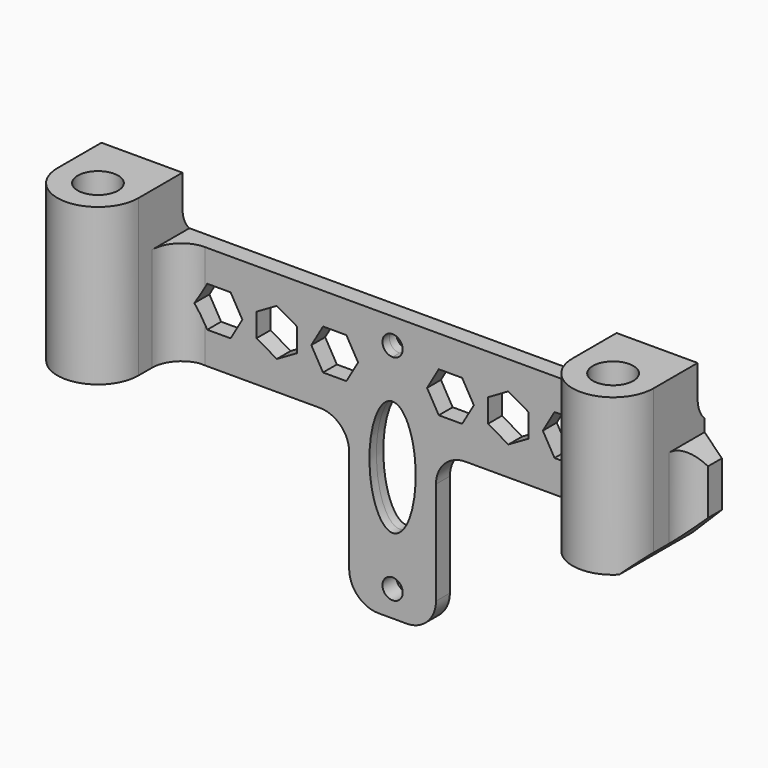
from build123d import *

# Parameters (mm, degrees)
F1_DEPTH      = 1.5
F2_R          = 3.5
F3_DEPTH      = 9
F4_DEPTH      = 9
F5_W          = 7.5
F5_H          = 37
F6_DEPTH      = 1.5
F8_DEPTH      = 12.7
F9_T1_DEPTH   = 3
F9_T3_DEPTH   = 17.9406090155
F9_T5_DEPTH   = 17.9406090155
F9_T7_DEPTH   = 17.9406090155
F9_T9_DEPTH   = 17.9406090155
F9_T11_DEPTH  = 14
F9_T13_DEPTH  = 14
F9_T15_DEPTH  = 3
F9_T17_DEPTH  = 28.4
F9_T19_DEPTH  = 28.4
F10_T1_DEPTH  = 29.1282991577
F10_T6_DEPTH  = 29.1282991577
F10_T11_DEPTH = 29.1282991577
F12_DEPTH     = 5.0038


# Not quite as in the source:
# - a fillet or chamfer that OpenCascade refuses, or shapes differently, is made with other operations: its cross-section is extruded or revolved along the edge and cut away or added


with BuildPart() as f1:
    # F0 (on Front) → F1 (new body, symmetric)
    with BuildSketch(Plane.XZ):
        Polygon((-54.5, 8.9406090155), (-54.5, -0.0593909845), (-54.5, -9.0593909845), (0, -9.0593909845), (0, 8.9406090155), align=None)
        Polygon((54.5, 8.9406090155), (0, 8.9406090155), (0, -9.0593909845), (54.5, -9.0593909845), (54.5, -0.0593909845), align=None)
    extrude(amount=F1_DEPTH, both=True)

    # F2 (on Top) → F3 (join, symmetric)
    with BuildSketch(Plane.XY):
        with BuildLine():
            ThreePointArc((-51.5, -9.5), (-44.5, -16.5), (-37.5, -9.5))
            ThreePointArc((-37.5, -9.5), (-44.5, -2.5), (-51.5, -9.5))
        make_face()
        with Locations((-44.5, -9.5)):
            Circle(F2_R, mode=Mode.SUBTRACT)
        with BuildLine():
            ThreePointArc((-51.5, -9.5), (-44.5, -2.5), (-37.5, -9.5))
            Line((-37.5, -9.5), (-37.5, 0))
            Line((-37.5, 0), (-51.5, 0))
            Line((-51.5, 0), (-51.5, -9.5))
        make_face()
        with BuildLine():
            Line((37.5, 0), (37.5, -9.5))
            ThreePointArc((37.5, -9.5), (44.5, -2.5), (51.5, -9.5))
            Line((51.5, -9.5), (51.5, 0))
            Line((51.5, 0), (37.5, 0))
        make_face()
        with BuildLine():
            ThreePointArc((51.5, -9.5), (44.5, -2.5), (37.5, -9.5))
            ThreePointArc((37.5, -9.5), (44.5, -16.5), (51.5, -9.5))
        make_face()
        with Locations((44.5, -9.5)):
            Circle(F2_R, mode=Mode.SUBTRACT)
    extrude(amount=F3_DEPTH, both=True)

    # F4 (add): faces of the model
    f4_faces = [f1.faces().sort_by_distance(p)[0] for p in [
        (-44.5, -16.2836091499, 9),
        (37.7163908501, -4.75, 9),
    ]]
    extrude(f4_faces, amount=F4_DEPTH)

    # F5 (on Front) → F6 (join, symmetric)
    with BuildSketch(Plane.XZ):
        with Locations((3.75, -18.5)):
            Rectangle(F5_W, F5_H)
        with Locations((-3.75, -18.5)):
            Rectangle(F5_W, F5_H)
    extrude(amount=F6_DEPTH, both=True)

    # F7 (on Front) → F8 (cut, symmetric)
    with BuildSketch(Plane.XZ):
        with BuildLine():
            ThreePointArc((1.75, -32.5), (1.2374368671, -31.2625631329), (0, -30.75))
            ThreePointArc((0, -30.75), (-1.2374368671, -33.7374368671), (1.75, -32.5))
        make_face()
        with BuildLine():
            add(Edge.make_bspline(
                [(0, -24), (4, -24), (4, -14), (4, -4), (0, -4)],
                knots=[0, 0, 0, 1.5707963268, 1.5707963268, 3.1415926536, 3.1415926536, 3.1415926536], degree=2, weights=[1, 0.7071067812, 1, 0.7071067812, 1]))
            Line((0, -4), (0, -14))
            Line((0, -14), (0, -24))
        make_face()
        with BuildLine():
            Line((0, -14), (0, -4))
            add(Edge.make_bspline(
                [(0, -4), (-4, -4), (-4, -14), (-4, -24), (0, -24)],
                knots=[3.1415926536, 3.1415926536, 3.1415926536, 4.7123889804, 4.7123889804, 6.2831853072, 6.2831853072, 6.2831853072], degree=2, weights=[1, 0.7071067812, 1, 0.7071067812, 1]))
            Line((0, -24), (0, -14))
        make_face()
        with BuildLine():
            ThreePointArc((1.75, 4.5), (-1.2374368671, 5.7374368671), (0, 2.75))
            ThreePointArc((0, 2.75), (1.2374368671, 3.2625631329), (1.75, 4.5))
        make_face()
    extrude(amount=F8_DEPTH, both=True, mode=Mode.SUBTRACT)

    # F9: fillet of radius 5.08 on 10 edges, made by hand

    # F9_s2 → F9_t1 (join)
    with BuildSketch(Plane.XZ.offset(-1.5)):
        with BuildLine():
            ThreePointArc((-12.58, -9.0593909845), (-8.9878975516, -10.547288536), (-7.5, -14.1393909845))
            Line((-7.5, -14.1393909845), (-7.3984, -14.1393909845))
            Line((-7.3984, -14.1393909845), (-7.3984, -8.9577909845))
            Line((-7.3984, -8.9577909845), (-12.58, -8.9577909845))
            Line((-12.58, -8.9577909845), (-12.58, -9.0593909845))
        make_face()
    extrude(amount=F9_T1_DEPTH)

    # F9_s4 → F9_t3 (join)
    with BuildSketch(Plane.XY.offset(-9)):
        with BuildLine():
            ThreePointArc((-54.5, -1.5), (-52.3154484409, -3.3742173421), (-51.5, -6.1346520905))
            Line((-51.5, -6.1346520905), (-51.3984, -6.1346520905))
            Line((-51.3984, -6.1346520905), (-51.3984, -1.5))
            Line((-51.3984, -1.5), (-51.5, -1.3984))
            ThreePointArc((-51.5, -1.3984), (-53, -1.3984), (-54.4584, -1.4073069582))
            Line((-54.4584, -1.4073069582), (-54.5, -1.5))
        make_face()
    extrude(amount=F9_T3_DEPTH)

    # F9_s6 → F9_t5 (join)
    with BuildSketch(Plane.XY.offset(-9)):
        with BuildLine():
            ThreePointArc((-32.42, -1.5), (-36.0121024484, -2.9878975516), (-37.5, -6.58))
            Line((-37.5, -6.58), (-37.6016, -6.58))
            Line((-37.6016, -6.58), (-37.6016, -1.3984))
            Line((-37.6016, -1.3984), (-32.42, -1.3984))
            Line((-32.42, -1.3984), (-32.42, -1.5))
        make_face()
    extrude(amount=F9_T5_DEPTH)

    # F9_s8 → F9_t7 (join)
    with BuildSketch(Plane.XY.offset(-9)):
        with BuildLine():
            ThreePointArc((32.42, -1.5), (36.0121024484, -2.9878975516), (37.5, -6.58))
            Line((37.5, -6.58), (37.6016, -6.58))
            Line((37.6016, -6.58), (37.6016, -1.3984))
            Line((37.6016, -1.3984), (32.42, -1.3984))
            Line((32.42, -1.3984), (32.42, -1.5))
        make_face()
    extrude(amount=F9_T7_DEPTH)

    # F9_s10 → F9_t9 (join)
    with BuildSketch(Plane.XY.offset(-9)):
        with BuildLine():
            ThreePointArc((54.5, -1.5), (52.3154484409, -3.3742173421), (51.5, -6.1346520905))
            Line((51.5, -6.1346520905), (51.3984, -6.1346520905))
            Line((51.3984, -6.1346520905), (51.3984, -1.5))
            Line((51.3984, -1.5), (51.5, -1.3984))
            ThreePointArc((51.5, -1.3984), (53, -1.3984), (54.4584, -1.4073069582))
            Line((54.4584, -1.4073069582), (54.5, -1.5))
        make_face()
    extrude(amount=F9_T9_DEPTH)

    # F9_s12 → F9_t11 (join)
    with BuildSketch(Plane.YZ.offset(37.5)):
        with BuildLine():
            ThreePointArc((1.5, 8.9406090155), (0.3899680172, 10.5928511441), (0, 12.5447732737))
            Line((0, 12.5447732737), (-0.1016, 12.5447732737))
            Line((-0.1016, 12.5447732737), (-0.1016, 8.9406090155))
            Line((-0.1016, 8.9406090155), (0, 8.8390090155))
            ThreePointArc((0, 8.8390090155), (0.75, 8.8390090155), (1.4284, 8.8685257304))
            Line((1.4284, 8.8685257304), (1.5, 8.9406090155))
        make_face()
    extrude(amount=F9_T11_DEPTH)

    # F9_s14 → F9_t13 (join)
    with BuildSketch(Plane.YZ.offset(-51.5)):
        with BuildLine():
            ThreePointArc((1.5, 8.9406090155), (0.3899680172, 10.5928511441), (0, 12.5447732737))
            Line((0, 12.5447732737), (-0.1016, 12.5447732737))
            Line((-0.1016, 12.5447732737), (-0.1016, 8.9406090155))
            Line((-0.1016, 8.9406090155), (0, 8.8390090155))
            ThreePointArc((0, 8.8390090155), (0.75, 8.8390090155), (1.4284, 8.8685257304))
            Line((1.4284, 8.8685257304), (1.5, 8.9406090155))
        make_face()
    extrude(amount=F9_T13_DEPTH)

    # F9_s16 → F9_t15 (join)
    with BuildSketch(Plane.XZ.offset(-1.5)):
        with BuildLine():
            ThreePointArc((12.58, -9.0593909845), (8.9878975516, -10.547288536), (7.5, -14.1393909845))
            Line((7.5, -14.1393909845), (7.3984, -14.1393909845))
            Line((7.3984, -14.1393909845), (7.3984, -8.9577909845))
            Line((7.3984, -8.9577909845), (12.58, -8.9577909845))
            Line((12.58, -8.9577909845), (12.58, -9.0593909845))
        make_face()
    extrude(amount=F9_T15_DEPTH)

    # F9_s18 → F9_t17 (cut)
    with BuildSketch(Plane.XZ.offset(-14.2)):
        with BuildLine():
            ThreePointArc((7.5, -31.92), (6.0121024484, -35.5121024484), (2.42, -37))
            Line((2.42, -37), (2.42, -37.1016))
            Line((2.42, -37.1016), (7.6016, -37.1016))
            Line((7.6016, -37.1016), (7.6016, -31.92))
            Line((7.6016, -31.92), (7.5, -31.92))
        make_face()
    extrude(amount=F9_T17_DEPTH, mode=Mode.SUBTRACT)

    # F9_s20 → F9_t19 (cut)
    with BuildSketch(Plane.XZ.offset(-14.2)):
        with BuildLine():
            ThreePointArc((-2.42, -37), (-6.0121024484, -35.5121024484), (-7.5, -31.92))
            Line((-7.5, -31.92), (-7.6016, -31.92))
            Line((-7.6016, -31.92), (-7.6016, -37.1016))
            Line((-7.6016, -37.1016), (-2.42, -37.1016))
            Line((-2.42, -37.1016), (-2.42, -37))
        make_face()
    extrude(amount=F9_T19_DEPTH, mode=Mode.SUBTRACT)

    # F10: chamfer of 5.08 on 4 edges, made by hand

    # F10_s2 → F10_t1 (cut)
    with BuildSketch(Plane.XZ.offset(-14.5641495789)):
        Polygon((-54.5, -3.9793909845), (-49.42, -9.0593909845), (-54.5, -9.0593909845), align=None)
        Polygon((54.5, -3.9793909845), (49.42, -9.0593909845), (54.5, -9.0593909845), align=None)
    extrude(amount=F10_T1_DEPTH, mode=Mode.SUBTRACT)


with BuildPart() as f10_tool4:
    # F10_s5 → F10_t6 (new body)
    with BuildSketch(Plane.XZ.offset(14.5641495789)):
        Polygon((-54.5, 3.8606090155), (-49.42, 8.9406090155), (-54.5, 8.9406090155), align=None)
    extrude(amount=-F10_T6_DEPTH)

    split(bisect_by=Plane.YZ.offset(-51.5), keep=Keep.BOTTOM)


with BuildPart() as f1_1:
    add(f1.part)

    # F10_t3: cut F10_tool4
    add(f10_tool4.part, mode=Mode.SUBTRACT)


with BuildPart() as f10_tool9:
    # F10_s10 → F10_t11 (new body)
    with BuildSketch(Plane.XZ.offset(14.5641495789)):
        Polygon((49.42, 8.9406090155), (54.5, 3.8606090155), (54.5, 8.9406090155), align=None)
    extrude(amount=-F10_T11_DEPTH)

    split(bisect_by=Plane.YZ.offset(51.5), keep=Keep.TOP)


with BuildPart() as f1_2:
    add(f1_1.part)

    # F10_t8: cut F10_tool9
    add(f10_tool9.part, mode=Mode.SUBTRACT)

    # F11 (on Front) → F12 (cut, symmetric)
    with BuildSketch(Plane.XZ):
        Polygon((-7.9792740578, -3.5), (-5.9585481157, 0), (-10, 0), (-14.0414518843, 0), (-12.0207259422, -3.5), align=None)
        Polygon((-10, 0), (-5.9585481157, 0), (-7.9792740578, 3.5), (-12.0207259422, 3.5), (-14.0414518843, 0), align=None)
        Polygon((-27.9792740578, -3.5), (-25.9585481157, 0), (-27.9792740578, 3.5), (-32.0207259422, 3.5), (-34.0414518843, 0), (-32.0207259422, -3.5), align=None)
        Polygon((-16.5, -2.0207259422), (-16.5, 0), (-20, 0), (-23.5, 0), (-23.5, -2.0207259422), (-20, -4.0414518843), align=None)
        Polygon((-20, 0), (-16.5, 0), (-16.5, 2.0207259422), (-20, 4.0414518843), (-23.5, 2.0207259422), (-23.5, 0), align=None)
        Polygon((34.0414518843, 0), (32.0207259422, 3.5), (27.9792740578, 3.5), (25.9585481157, 0), (27.9792740578, -3.5), (32.0207259422, -3.5), align=None)
        Polygon((20, -4.0414518843), (23.5, -2.0207259422), (23.5, 2.0207259422), (20, 4.0414518843), (16.5, 2.0207259422), (16.5, -2.0207259422), align=None)
        Polygon((14.0414518843, 0), (12.0207259422, 3.5), (7.9792740578, 3.5), (5.9585481157, 0), (7.9792740578, -3.5), (12.0207259422, -3.5), align=None)
    extrude(amount=F12_DEPTH, both=True, mode=Mode.SUBTRACT)


solid = f1_2.part
